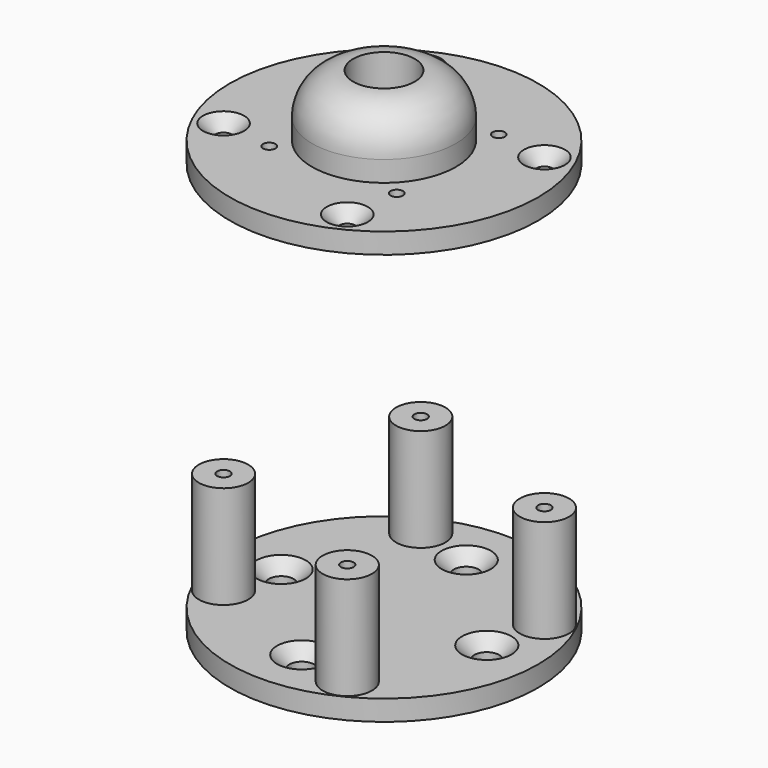
from build123d import *

# Parameters (mm, degrees)
F0_R      = 37.5
F0_R_2    = 6
F0_R_3    = 3
F0_R_4    = 1.55
F1_DEPTH  = 5
F2_SIZE   = 3
F4_R      = 37.5
F4_R_2    = 2
F4_R_3    = 1.5
F5_DEPTH  = 5
F6_DEPTH  = 5
F7_DEPTH  = 30
F8_DEPTH  = 2.5
F9_SIZE   = 3
F10_R     = 17.5
F10_R_2   = 7.5
F11_DEPTH = 15
F12_R     = 9.99999


# Not quite as in the source:
# - a fillet or chamfer is up to 0.001 mm smaller than in the source, because OpenCascade refuses the exact size


with BuildPart() as f1:
    # F0 (on Top) → F1 (new body)
    with BuildSketch(Plane.XY):
        Circle(F0_R)
        with Locations((-28.15, -13.5888777375)):
            Circle(F0_R_2, mode=Mode.SUBTRACT)
        with Locations((13.5888777375, -28.15)):
            Circle(F0_R_2, mode=Mode.SUBTRACT)
        with Locations((0, -25)):
            Circle(F0_R_3, mode=Mode.SUBTRACT)
        with Locations((-25, 0)):
            Circle(F0_R_3, mode=Mode.SUBTRACT)
        with Locations((-13.5888777375, 28.15)):
            Circle(F0_R_2, mode=Mode.SUBTRACT)
        with Locations((25, 0)):
            Circle(F0_R_3, mode=Mode.SUBTRACT)
        with Locations((28.15, 13.5888777375)):
            Circle(F0_R_2, mode=Mode.SUBTRACT)
        with Locations((0, 25)):
            Circle(F0_R_3, mode=Mode.SUBTRACT)
        with Locations((28.15, 13.5888777375)):
            Circle(F0_R_2)
        Polygon((31.0096664331, 14.9693273833), (30.7753376785, 11.802558783), (27.9156712454, 10.4221091372), (25.2903335669, 12.2084280917), (25.5246623215, 15.375196692), (28.3843287546, 16.7556463378), align=None, mode=Mode.SUBTRACT)
        with Locations((-28.15, -13.5888777375)):
            Circle(F0_R_2)
        Polygon((-25.5246623215, -15.375196692), (-28.3843287546, -16.7556463378), (-31.0096664331, -14.9693273833), (-30.7753376785, -11.802558783), (-27.9156712454, -10.4221091372), (-25.2903335669, -12.2084280917), align=None, mode=Mode.SUBTRACT)
        with Locations((-13.5888777375, 28.15)):
            Circle(F0_R_2)
        Polygon((-15.375196692, 25.5246623215), (-16.7556463378, 28.3843287546), (-14.9693273833, 31.0096664331), (-11.802558783, 30.7753376785), (-10.4221091372, 27.9156712454), (-12.2084280917, 25.2903335669), align=None, mode=Mode.SUBTRACT)
        with Locations((13.5888777375, -28.15)):
            Circle(F0_R_2)
        Polygon((15.375196692, -25.5246623215), (16.7556463378, -28.3843287546), (14.9693273833, -31.0096664331), (11.802558783, -30.7753376785), (10.4221091372, -27.9156712454), (12.2084280917, -25.2903335669), align=None, mode=Mode.SUBTRACT)
        Polygon((-14.9693273833, 31.0096664331), (-16.7556463378, 28.3843287546), (-15.375196692, 25.5246623215), (-12.2084280917, 25.2903335669), (-10.4221091372, 27.9156712454), (-11.802558783, 30.7753376785), align=None)
        with Locations((-13.5888777375, 28.15)):
            Circle(F0_R_4, mode=Mode.SUBTRACT)
        Polygon((14.9693273833, -31.0096664331), (16.7556463378, -28.3843287546), (15.375196692, -25.5246623215), (12.2084280917, -25.2903335669), (10.4221091372, -27.9156712454), (11.802558783, -30.7753376785), align=None)
        with Locations((13.5888777375, -28.15)):
            Circle(F0_R_4, mode=Mode.SUBTRACT)
        Polygon((-31.0096664331, -14.9693273833), (-28.3843287546, -16.7556463378), (-25.5246623215, -15.375196692), (-25.2903335669, -12.2084280917), (-27.9156712454, -10.4221091372), (-30.7753376785, -11.802558783), align=None)
        with Locations((-28.15, -13.5888777375)):
            Circle(F0_R_4, mode=Mode.SUBTRACT)
        Polygon((27.9156712454, 10.4221091372), (30.7753376785, 11.802558783), (31.0096664331, 14.9693273833), (28.3843287546, 16.7556463378), (25.5246623215, 15.375196692), (25.2903335669, 12.2084280917), align=None)
        with Locations((28.15, 13.5888777375)):
            Circle(F0_R_4, mode=Mode.SUBTRACT)
    extrude(amount=F1_DEPTH)

    # F2
    f2_edges = [f1.edges().sort_by_distance(p)[0] for p in [
        (-3, 25, 5),
        (22, 0, 5),
        (-3, -25, 5),
        (-28, 0, 5),
    ]]
    chamfer(f2_edges, length=F2_SIZE)

    # F0 (on Top) → F7 (join)
    with BuildSketch(Plane.XY):
        with Locations((28.15, 13.5888777375)):
            Circle(F0_R_2)
        Polygon((31.0096664331, 14.9693273833), (30.7753376785, 11.802558783), (27.9156712454, 10.4221091372), (25.2903335669, 12.2084280917), (25.5246623215, 15.375196692), (28.3843287546, 16.7556463378), align=None, mode=Mode.SUBTRACT)
        Polygon((27.9156712454, 10.4221091372), (30.7753376785, 11.802558783), (31.0096664331, 14.9693273833), (28.3843287546, 16.7556463378), (25.5246623215, 15.375196692), (25.2903335669, 12.2084280917), align=None)
        with Locations((28.15, 13.5888777375)):
            Circle(F0_R_4, mode=Mode.SUBTRACT)
        with Locations((-13.5888777375, 28.15)):
            Circle(F0_R_2)
        Polygon((-15.375196692, 25.5246623215), (-16.7556463378, 28.3843287546), (-14.9693273833, 31.0096664331), (-11.802558783, 30.7753376785), (-10.4221091372, 27.9156712454), (-12.2084280917, 25.2903335669), align=None, mode=Mode.SUBTRACT)
        Polygon((-14.9693273833, 31.0096664331), (-16.7556463378, 28.3843287546), (-15.375196692, 25.5246623215), (-12.2084280917, 25.2903335669), (-10.4221091372, 27.9156712454), (-11.802558783, 30.7753376785), align=None)
        with Locations((-13.5888777375, 28.15)):
            Circle(F0_R_4, mode=Mode.SUBTRACT)
        with Locations((-28.15, -13.5888777375)):
            Circle(F0_R_2)
        Polygon((-25.5246623215, -15.375196692), (-28.3843287546, -16.7556463378), (-31.0096664331, -14.9693273833), (-30.7753376785, -11.802558783), (-27.9156712454, -10.4221091372), (-25.2903335669, -12.2084280917), align=None, mode=Mode.SUBTRACT)
        Polygon((-31.0096664331, -14.9693273833), (-28.3843287546, -16.7556463378), (-25.5246623215, -15.375196692), (-25.2903335669, -12.2084280917), (-27.9156712454, -10.4221091372), (-30.7753376785, -11.802558783), align=None)
        with Locations((-28.15, -13.5888777375)):
            Circle(F0_R_4, mode=Mode.SUBTRACT)
        with Locations((13.5888777375, -28.15)):
            Circle(F0_R_2)
        Polygon((15.375196692, -25.5246623215), (16.7556463378, -28.3843287546), (14.9693273833, -31.0096664331), (11.802558783, -30.7753376785), (10.4221091372, -27.9156712454), (12.2084280917, -25.2903335669), align=None, mode=Mode.SUBTRACT)
        Polygon((14.9693273833, -31.0096664331), (16.7556463378, -28.3843287546), (15.375196692, -25.5246623215), (12.2084280917, -25.2903335669), (10.4221091372, -27.9156712454), (11.802558783, -30.7753376785), align=None)
        with Locations((13.5888777375, -28.15)):
            Circle(F0_R_4, mode=Mode.SUBTRACT)
    extrude(amount=F7_DEPTH)

    # F0 (on Top) → F8 (cut)
    with BuildSketch(Plane.XY):
        Polygon((-31.0096664331, -14.9693273833), (-28.3843287546, -16.7556463378), (-25.5246623215, -15.375196692), (-25.2903335669, -12.2084280917), (-27.9156712454, -10.4221091372), (-30.7753376785, -11.802558783), align=None)
        with Locations((-28.15, -13.5888777375)):
            Circle(F0_R_4, mode=Mode.SUBTRACT)
        Polygon((-14.9693273833, 31.0096664331), (-16.7556463378, 28.3843287546), (-15.375196692, 25.5246623215), (-12.2084280917, 25.2903335669), (-10.4221091372, 27.9156712454), (-11.802558783, 30.7753376785), align=None)
        with Locations((-13.5888777375, 28.15)):
            Circle(F0_R_4, mode=Mode.SUBTRACT)
        Polygon((27.9156712454, 10.4221091372), (30.7753376785, 11.802558783), (31.0096664331, 14.9693273833), (28.3843287546, 16.7556463378), (25.5246623215, 15.375196692), (25.2903335669, 12.2084280917), align=None)
        with Locations((28.15, 13.5888777375)):
            Circle(F0_R_4, mode=Mode.SUBTRACT)
        Polygon((14.9693273833, -31.0096664331), (16.7556463378, -28.3843287546), (15.375196692, -25.5246623215), (12.2084280917, -25.2903335669), (10.4221091372, -27.9156712454), (11.802558783, -30.7753376785), align=None)
        with Locations((13.5888777375, -28.15)):
            Circle(F0_R_4, mode=Mode.SUBTRACT)
    extrude(amount=F8_DEPTH, mode=Mode.SUBTRACT)


with BuildPart() as f5:
    # F4 (on offset) → F5 (new body)
    with BuildSketch(Plane.XY.offset(100)):
        Circle(F4_R)
        with Locations((-28.15, -13.5888777375)):
            Circle(F4_R_2, mode=Mode.SUBTRACT)
        with Locations((-15.5, -15.5)):
            Circle(F4_R_3, mode=Mode.SUBTRACT)
        with Locations((13.5888777375, -28.15)):
            Circle(F4_R_2, mode=Mode.SUBTRACT)
        with BuildLine():
            ThreePointArc((17, -15.5), (15.5, -17), (14, -15.5))
            ThreePointArc((14, -15.5), (15.5, -14), (17, -15.5))
        make_face(mode=Mode.SUBTRACT)
        with Locations((-15.5, 15.5)):
            Circle(F4_R_3, mode=Mode.SUBTRACT)
        with Locations((-13.5888777375, 28.15)):
            Circle(F4_R_2, mode=Mode.SUBTRACT)
        with BuildLine():
            ThreePointArc((6, 0), (4.2426406871, -4.2426406871), (0, -6))
            ThreePointArc((0, -6), (-4.2426406871, 4.2426406871), (6, 0))
        make_face(mode=Mode.SUBTRACT)
        with Locations((15.5, 15.5)):
            Circle(F4_R_3, mode=Mode.SUBTRACT)
        with Locations((28.15, 13.5888777375)):
            Circle(F4_R_2, mode=Mode.SUBTRACT)
    extrude(amount=F5_DEPTH)

    # F4 (on offset) → F6 (join)
    with BuildSketch(Plane.XY.offset(100)):
        Circle(F4_R)
        with Locations((-28.15, -13.5888777375)):
            Circle(F4_R_2, mode=Mode.SUBTRACT)
        with Locations((-15.5, -15.5)):
            Circle(F4_R_3, mode=Mode.SUBTRACT)
        with Locations((13.5888777375, -28.15)):
            Circle(F4_R_2, mode=Mode.SUBTRACT)
        with BuildLine():
            ThreePointArc((17, -15.5), (15.5, -17), (14, -15.5))
            ThreePointArc((14, -15.5), (15.5, -14), (17, -15.5))
        make_face(mode=Mode.SUBTRACT)
        with Locations((-15.5, 15.5)):
            Circle(F4_R_3, mode=Mode.SUBTRACT)
        with Locations((-13.5888777375, 28.15)):
            Circle(F4_R_2, mode=Mode.SUBTRACT)
        with BuildLine():
            ThreePointArc((6, 0), (4.2426406871, -4.2426406871), (0, -6))
            ThreePointArc((0, -6), (-4.2426406871, 4.2426406871), (6, 0))
        make_face(mode=Mode.SUBTRACT)
        with Locations((15.5, 15.5)):
            Circle(F4_R_3, mode=Mode.SUBTRACT)
        with Locations((28.15, 13.5888777375)):
            Circle(F4_R_2, mode=Mode.SUBTRACT)
    extrude(amount=F6_DEPTH)

    # F9
    f9_edges = [f5.edges().sort_by_distance(p)[0] for p in [
        (-30.15, -13.588878, 105),
        (-15.588878, 28.15, 105),
        (26.15, 13.588878, 105),
        (11.588878, -28.15, 105),
    ]]
    chamfer(f9_edges, length=F9_SIZE)

    # F10 (on face) → F11 (join)
    with BuildSketch(Plane.XY.offset(105)):
        Circle(F10_R)
        Circle(F10_R_2, mode=Mode.SUBTRACT)
    extrude(amount=F11_DEPTH)

    # F12 (radius 10 in the source; OpenCascade refuses exactly that, so slightly less here)
    f12_edges = [f5.edges().sort_by_distance(p)[0] for p in [
        (-17.5, 0, 120),
    ]]
    fillet(f12_edges, radius=F12_R)


solid = Compound([f1.part, f5.part])
